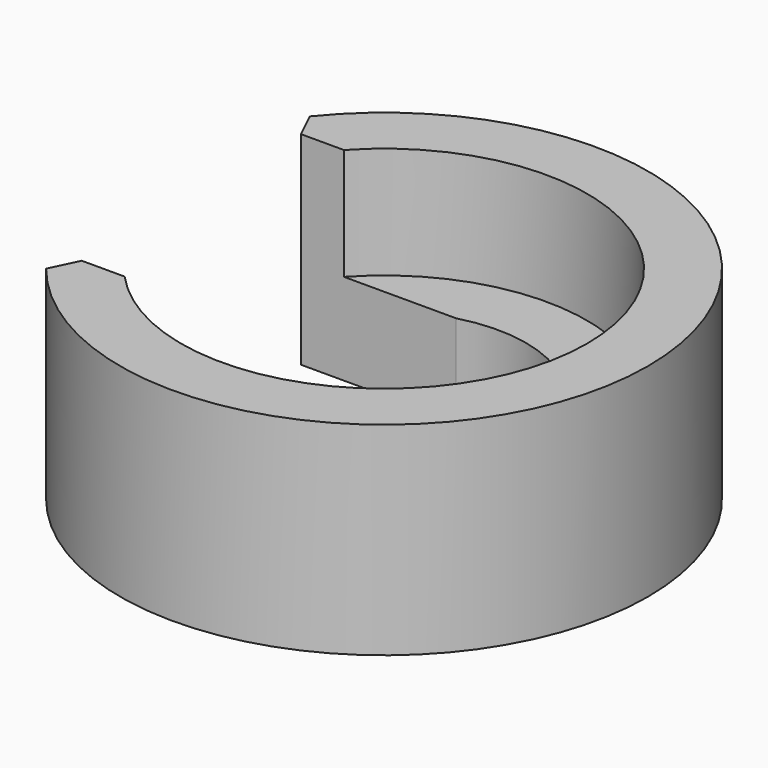
from build123d import *

# Parameters (mm, degrees)
F0_R        = 13
F0_R_2      = 7
F1_DEPTH    = 10
F2_R        = 10
F2_R_2      = 7
F3_DEPTH    = 5.5
F4_W        = 13.5
F4_H        = 13.5
F5_DEPTH    = 10.001
F6_T1_DEPTH = 18.5160584479


# Not quite as in the source:
# - a fillet or chamfer that OpenCascade refuses, or shapes differently, is made with other operations: its cross-section is extruded or revolved along the edge and cut away or added


with BuildPart() as f1:
    # F0 (on Top) → F1 (new body)
    with BuildSketch(Plane.XY):
        Circle(F0_R)
        Circle(F0_R_2, mode=Mode.SUBTRACT)
    extrude(amount=F1_DEPTH)

    # F2 (on face) → F3 (cut)
    with BuildSketch(Plane.XY.offset(10)):
        Circle(F2_R)
        Circle(F2_R_2, mode=Mode.SUBTRACT)
    extrude(amount=-F3_DEPTH, mode=Mode.SUBTRACT)

    # F4 (on face) → F5 (cut, through all)
    with BuildSketch(Plane.XY.offset(10)):
        with Locations((-6.75, 0)):
            Rectangle(F4_W, F4_H)
    extrude(amount=-F5_DEPTH, mode=Mode.SUBTRACT)

    # F6: chamfer of 1.5 on 2 edges, made by hand

    # F6_s2 → F6_t1 (cut)
    with BuildSketch(Plane.XY.offset(-4.2580292239)):
        with BuildLine():
            Line((-10.1773648706, 8.1750152332), (-9.4664670488, 6.6959219319))
            Line((-9.4664670488, 6.6959219319), (-9.4664670488, 6.6659219319))
            ThreePointArc((-9.4664670488, 6.6659219319), (-10.2883550352, 6.72), (-11.1102430216, 6.72))
            Line((-11.1102430216, 6.72), (-11.135882044, 6.7655769231))
            ThreePointArc((-11.135882044, 6.7655769231), (-10.669011075, 7.4801806583), (-10.2007911166, 8.1937558574))
            Line((-10.2007911166, 8.1937558574), (-10.1773648706, 8.1750152332))
        make_face()
        with BuildLine():
            Line((-10.1773648706, -8.1750152332), (-9.4664670488, -6.6959219319))
            Line((-9.4664670488, -6.6959219319), (-9.4664670488, -6.6659219319))
            ThreePointArc((-9.4664670488, -6.6659219319), (-10.2883550352, -6.72), (-11.1102430216, -6.72))
            Line((-11.1102430216, -6.72), (-11.135882044, -6.7655769231))
            ThreePointArc((-11.135882044, -6.7655769231), (-10.669011075, -7.4801806583), (-10.2007911166, -8.1937558574))
            Line((-10.2007911166, -8.1937558574), (-10.1773648706, -8.1750152332))
        make_face()
    extrude(amount=F6_T1_DEPTH, mode=Mode.SUBTRACT)


solid = f1.part
